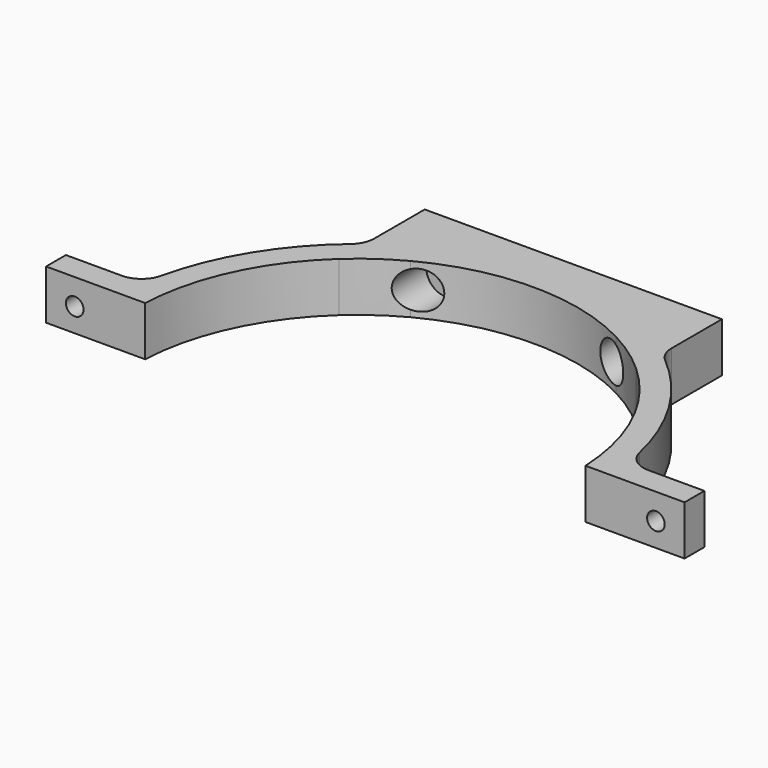
from build123d import *
from build123d import SkipClean  # not in build123d's __all__

# Parameters (mm, degrees)
F1_DEPTH       = 10
F3_D           = 3.556
F3_CBORE_D     = 7.62
F3_CBORE_DEPTH = 13.75
F4_DEPTH       = 10.0010001
F6_D           = 3.556
F7_R           = 5


with BuildPart() as f1:
    # F0 (on Top) → F1 (new body)
    with BuildSketch(Plane.XY):
        with BuildLine():
            ThreePointArc((30, 32.8671568591), (40.2999174323, 18.8723780946), (44.4550334608, 2))
            Line((44.4550334608, 2), (44.4550334608, 7))
            Line((44.4550334608, 7), (49.002550954, 7))
            ThreePointArc((49.002550954, 7), (42.6890737127, 25.0577929106), (30, 39.3732142452))
            Line((30, 39.3732142452), (30, 32.8671568591))
        make_face()
        with BuildLine():
            ThreePointArc((20.7364413533, 39.3732142452), (25.5759421328, 36.4159468368), (30, 32.8671568591))
            Line((30, 32.8671568591), (30, 39.3732142452))
            Line((30, 39.3732142452), (20.7364413533, 39.3732142452))
        make_face()
        with BuildLine():
            ThreePointArc((-20.7364413533, 39.3732142452), (0, 44.5), (20.7364413533, 39.3732142452))
            Line((20.7364413533, 39.3732142452), (30, 39.3732142452))
            ThreePointArc((30, 39.3732142452), (15.8315491079, 46.9000218853), (-1.83e-08, 49.5))
            ThreePointArc((-1.83e-08, 49.5), (-15.8315491253, 46.9000218795), (-30, 39.3732142452))
            Line((-30, 39.3732142452), (-20.7364413533, 39.3732142452))
        make_face()
        with BuildLine():
            Line((-30, 39.3732142452), (-30, 32.8671568591))
            ThreePointArc((-30, 32.8671568591), (-25.5759421328, 36.4159468368), (-20.7364413533, 39.3732142452))
            Line((-20.7364413533, 39.3732142452), (-30, 39.3732142452))
        make_face()
        with BuildLine():
            ThreePointArc((-44.4550334608, 2), (-40.2999174323, 18.8723780946), (-30, 32.8671568591))
            Line((-30, 32.8671568591), (-30, 39.3732142452))
            ThreePointArc((-30, 39.3732142452), (-42.6890737127, 25.0577929106), (-49.002550954, 7))
            Line((-49.002550954, 7), (-44.4550334608, 7))
            Line((-44.4550334608, 7), (-44.4550334608, 2))
        make_face()
        with BuildLine():
            Line((-64.4550334608, 2), (-49.4595794564, 2))
            ThreePointArc((-49.4595794564, 2), (-49.2945005172, 4.5057983491), (-49.002550954, 7))
            Line((-49.002550954, 7), (-64.4550334608, 7))
            Line((-64.4550334608, 7), (-64.4550334608, 2))
        make_face()
        with BuildLine():
            Line((-49.4595794564, 2), (-44.4550334608, 2))
            Line((-44.4550334608, 2), (-44.4550334608, 7))
            Line((-44.4550334608, 7), (-49.002550954, 7))
            ThreePointArc((-49.002550954, 7), (-49.2945005172, 4.5057983491), (-49.4595794564, 2))
        make_face()
        with BuildLine():
            Line((44.4550334608, 7), (44.4550334608, 2))
            Line((44.4550334608, 2), (49.4595794564, 2))
            ThreePointArc((49.4595794564, 2), (49.2945005172, 4.5057983491), (49.002550954, 7))
            Line((49.002550954, 7), (44.4550334608, 7))
        make_face()
        with BuildLine():
            ThreePointArc((49.002550954, 7), (49.2945005172, 4.5057983491), (49.4595794564, 2))
            Line((49.4595794564, 2), (64.4550334608, 2))
            Line((64.4550334608, 2), (64.4550334608, 7))
            Line((64.4550334608, 7), (49.002550954, 7))
        make_face()
        with BuildLine():
            Line((-30, 49.5), (-30, 39.3732142452))
            ThreePointArc((-30, 39.3732142452), (-15.8315491253, 46.9000218795), (-1.83e-08, 49.5))
            Line((-1.83e-08, 49.5), (-30, 49.5))
        make_face()
        with BuildLine():
            ThreePointArc((-1.83e-08, 49.5), (15.8315491079, 46.9000218853), (30, 39.3732142452))
            Line((30, 39.3732142452), (30, 49.5))
            Line((30, 49.5), (-1.83e-08, 49.5))
        make_face()
        with BuildLine():
            Line((-30, 32.8671568591), (30, 32.8671568591))
            ThreePointArc((30, 32.8671568591), (25.5759421328, 36.4159468368), (20.7364413533, 39.3732142452))
            Line((20.7364413533, 39.3732142452), (-20.7364413533, 39.3732142452))
            ThreePointArc((-20.7364413533, 39.3732142452), (-25.5759421328, 36.4159468368), (-30, 32.8671568591))
        make_face()
        Polygon((-30, 49.5), (-1.83e-08, 49.5), (30, 49.5), (30, 54.5), (-30, 54.5), align=None)
    extrude(amount=F1_DEPTH)

    # F3 (through all)
    with Locations(Plane.XZ.offset(-32.8671568591)):
        with Locations((-19.558, 4.9517820589), (19.558, 4.9517820589)):
            CounterBoreHole(F3_D / 2, F3_CBORE_D / 2, F3_CBORE_DEPTH)

    # F0 (on Top) → F4 (cut, through all)
    with BuildSketch(Plane.XY):
        with BuildLine():
            Line((-30, 32.8671568591), (30, 32.8671568591))
            ThreePointArc((30, 32.8671568591), (25.5759421328, 36.4159468368), (20.7364413533, 39.3732142452))
            Line((20.7364413533, 39.3732142452), (-20.7364413533, 39.3732142452))
            ThreePointArc((-20.7364413533, 39.3732142452), (-25.5759421328, 36.4159468368), (-30, 32.8671568591))
        make_face()
    with SkipClean():  # cleaning this boolean's faces spoils the solid; the shape is the same uncleaned
        extrude(amount=F4_DEPTH, mode=Mode.SUBTRACT)

    # F6 (through all)
    with Locations(Plane.XZ.offset(-2)):
        with Locations((-58.674, 4.78035165), (58.674, 4.78035165)):
            Hole(F6_D / 2)

    # F7
    f7_edges = [f1.edges().sort_by_distance(p)[0] for p in [
        (-49.002551, 7, 5),
        (49.002551, 7, 5),
        (30, 39.373214, 5),
        (-30, 39.373214, 5),
    ]]
    fillet(f7_edges, radius=F7_R)


solid = f1.part
